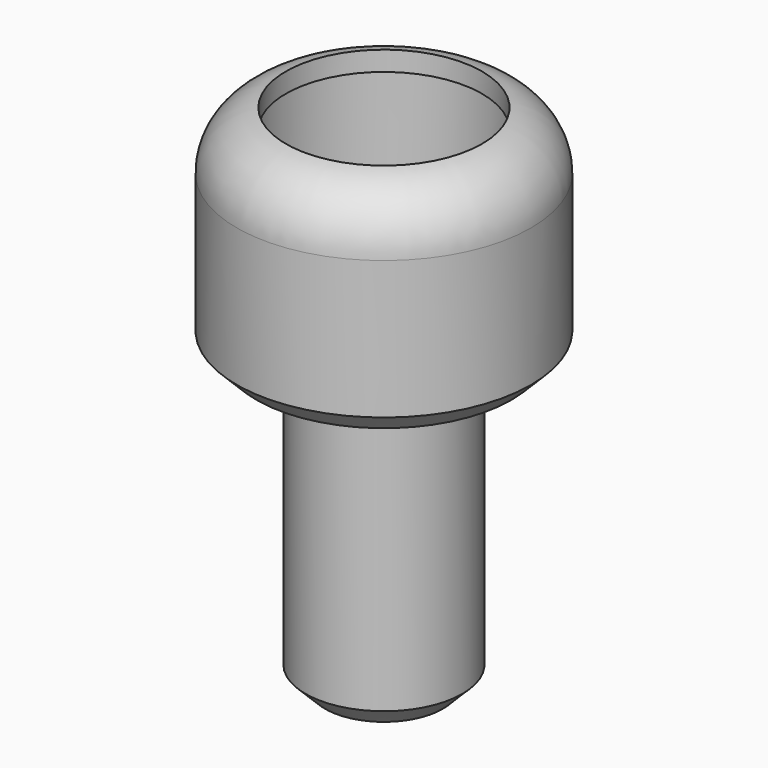
from build123d import *

# Parameters (mm, degrees)
F0_R     = 7.5
F1_DEPTH = 10
F2_R     = 4
F3_DEPTH = 15
F4_T     = -2
F5_R     = 7.5
F5_R_2   = 5
F6_DEPTH = 1
F8_SIZE  = 1
F9_SIZE  = 1


# Not quite as in the source:
# - a fillet or chamfer that OpenCascade refuses, or shapes differently, is made with other operations: its cross-section is extruded or revolved along the edge and cut away or added


with BuildPart() as f1:
    # F0 (on Top) → F1 (new body)
    with BuildSketch(Plane.XY):
        Circle(F0_R)
    extrude(amount=F1_DEPTH)

    # F2 (on face) → F3 (join)
    with BuildSketch(Plane(origin=(0, 0, 0), x_dir=(1, 0, 0), z_dir=(0, 0, -1))):
        Circle(F2_R)
    extrude(amount=F3_DEPTH)

    # F4
    f4_openings = [f1.faces().sort_by_distance(p)[0] for p in [
        (0, 0, 10),
        (0, 0, -15),
    ]]
    offset(amount=F4_T, openings=f4_openings, kind=Kind.INTERSECTION)

    # F5 (on face) → F6 (join)
    with BuildSketch(Plane.XY.offset(10)):
        Circle(F5_R)
        Circle(F5_R_2, mode=Mode.SUBTRACT)
    extrude(amount=F6_DEPTH)

    # F7: fillet of radius 3 on 1 edges, made by hand

    # F7_s1 → F7_t2 (revolve, cut)
    with BuildSketch(Plane.XZ):
        with BuildLine():
            ThreePointArc((7.5, 8.0419601084), (6.7912878475, 9.9784517816), (5, 11))
            Line((5, 11), (7.5, 11))
            Line((7.5, 11), (7.5, 8.0419601084))
        make_face()
    revolve(axis=Axis((0, 0, 11), (0, 0, 1)), mode=Mode.SUBTRACT)

    # F8
    f8_edges = [f1.edges().sort_by_distance(p)[0] for p in [
        (-7.5, 0, 0),
    ]]
    chamfer(f8_edges, length=F8_SIZE)

    # F9
    f9_edges = [f1.edges().sort_by_distance(p)[0] for p in [
        (-4, 0, -15),
    ]]
    chamfer(f9_edges, length=F9_SIZE)


solid = f1.part
